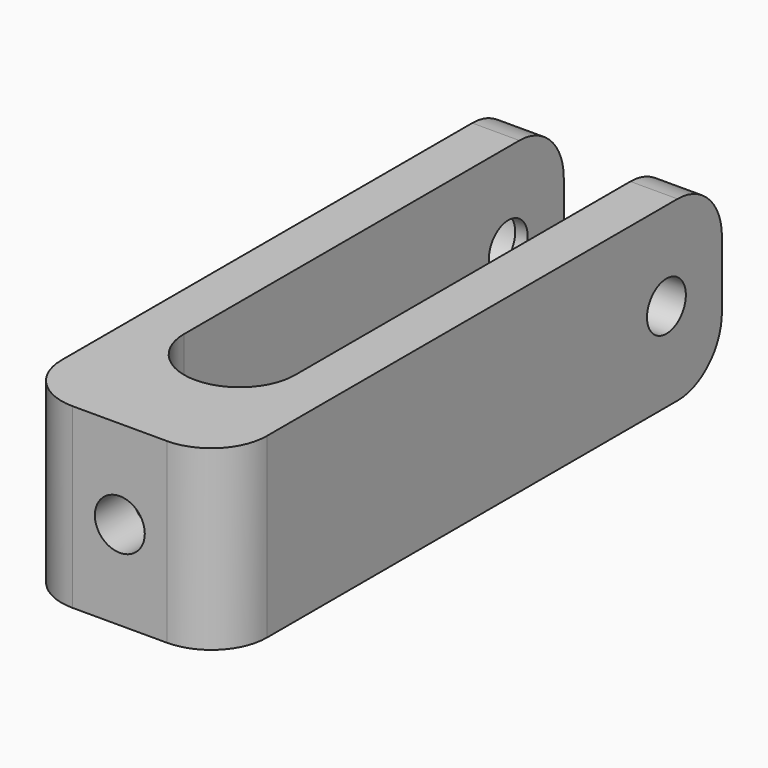
from build123d import *

# Parameters (mm, degrees)
F0_W         = 3.4
F0_H         = 12.8
F0_W_2       = 8
F0_R         = 1.8
F1_DEPTH     = 45
F2_R         = 1.75
F3_DEPTH     = 25
F2_R_2       = 3
F4_DEPTH     = 2.5
F0_H_2       = 0.6
F5_DEPTH     = 38.2
F6_T3_DEPTH  = 12.8
F6_S4_R      = 1.8
F6_T5_DEPTH  = 8
F6_T8_DEPTH  = 12.8
F6_S9_R      = 1.8
F6_T10_DEPTH = 8
F6_T14_DEPTH = 23.4
F6_T17_DEPTH = 23.4
F6_T20_DEPTH = 23.4
F6_T23_DEPTH = 23.4
F6_T26_DEPTH = 32.8
F6_T29_DEPTH = 32.8
F7_DEPTH     = 41.6


# Not quite as in the source:
# - a fillet or chamfer that OpenCascade refuses, or shapes differently, is made with other operations: its cross-section is extruded or revolved along the edge and cut away or added


with BuildPart() as f1:
    # F0 (on Front) → F1 (new body)
    with BuildSketch(Plane.XZ):
        with Locations((-1.7, 6.4)):
            Rectangle(F0_W, F0_H)
        with Locations((-7.4, 6.4)):
            Rectangle(F0_W_2, F0_H)
        Polygon((-10.8641016151, 6.4), (-9.1320508076, 9.4), (-5.6679491924, 9.4), (-3.9358983849, 6.4), (-5.6679491924, 3.4), (-9.1320508076, 3.4), align=None, mode=Mode.SUBTRACT)
        with Locations((-13.1, 6.4)):
            Rectangle(F0_W, F0_H)
        Polygon((-5.6679491924, 9.4), (-9.1320508076, 9.4), (-10.8641016151, 6.4), (-9.1320508076, 3.4), (-5.6679491924, 3.4), (-3.9358983849, 6.4), align=None)
        with Locations((-7.4, 6.4)):
            Circle(F0_R, mode=Mode.SUBTRACT)
    extrude(amount=F1_DEPTH)

    # F2 (on face) → F3 (cut)
    with BuildSketch(Plane(origin=(-14.8, 0, 0), x_dir=(0, -1, 0), z_dir=(-1, 0, 0))):
        with Locations((5, 6.4)):
            Circle(F2_R)
    extrude(amount=-F3_DEPTH, mode=Mode.SUBTRACT)

    # F2 (on face) → F4 (cut)
    with BuildSketch(Plane(origin=(-14.8, 0, 0), x_dir=(0, -1, 0), z_dir=(-1, 0, 0))):
        with Locations((5, 6.4)):
            Circle(F2_R_2)
        with Locations((5, 6.4)):
            Circle(F2_R, mode=Mode.SUBTRACT)
    extrude(amount=-F4_DEPTH, mode=Mode.SUBTRACT)

    # F0 (on Front) → F5 (cut)
    with BuildSketch(Plane.XZ):
        with Locations((-7.4, 13.1)):
            Rectangle(F0_W_2, F0_H_2)
        with Locations((-7.4, 6.4)):
            Rectangle(F0_W_2, F0_H)
        Polygon((-10.8641016151, 6.4), (-9.1320508076, 9.4), (-5.6679491924, 9.4), (-3.9358983849, 6.4), (-5.6679491924, 3.4), (-9.1320508076, 3.4), align=None, mode=Mode.SUBTRACT)
        with Locations((-7.4, -0.3)):
            Rectangle(F0_W_2, F0_H_2)
        Polygon((-5.6679491924, 9.4), (-9.1320508076, 9.4), (-10.8641016151, 6.4), (-9.1320508076, 3.4), (-5.6679491924, 3.4), (-3.9358983849, 6.4), align=None)
        with Locations((-7.4, 6.4)):
            Circle(F0_R, mode=Mode.SUBTRACT)
    extrude(amount=F5_DEPTH, mode=Mode.SUBTRACT)

    # F6: fillet of radius 4 on 8 edges, made by hand


with BuildPart() as f6_tool1:
    # F6_s2 → F6_t3 (new body)
    with BuildSketch(Plane.XY):
        with BuildLine():
            ThreePointArc((-7.4, -38.2), (-4.5715728753, -37.0284271247), (-3.4, -34.2))
            Line((-3.4, -34.2), (-3.4, -38.2))
            Line((-3.4, -38.2), (-7.4, -38.2))
        make_face()
    extrude(amount=F6_T3_DEPTH)

    # F6_s4 → F6_t5 (cut, symmetric)
    with BuildSketch(Plane.XZ.offset(36.2)):
        with Locations((-7.4, 6.4)):
            Circle(F6_S4_R)
    extrude(amount=F6_T5_DEPTH, both=True, mode=Mode.SUBTRACT)


with BuildPart() as f6_tool6:
    # F6_s7 → F6_t8 (new body)
    with BuildSketch(Plane.XY.offset(12.8)):
        with BuildLine():
            ThreePointArc((-11.4, -34.2), (-10.2284271247, -37.0284271247), (-7.4, -38.2))
            Line((-7.4, -38.2), (-11.4, -38.2))
            Line((-11.4, -38.2), (-11.4, -34.2))
        make_face()
    extrude(amount=-F6_T8_DEPTH)

    # F6_s9 → F6_t10 (cut, symmetric)
    with BuildSketch(Plane.XZ.offset(36.2)):
        with Locations((-7.4, 6.4)):
            Circle(F6_S9_R)
    extrude(amount=F6_T10_DEPTH, both=True, mode=Mode.SUBTRACT)


with BuildPart() as f1_1:
    add(f1.part)

    # F6_t11: union F6_tool1, F6_tool6
    add([f6_tool1.part, f6_tool6.part])


with BuildPart() as f6_tool12:
    # F6_s13 → F6_t14 (new body)
    with BuildSketch(Plane.YZ.offset(10)):
        with BuildLine():
            ThreePointArc((0, 8.8), (-1.1715728753, 11.6284271247), (-4, 12.8))
            Line((-4, 12.8), (0, 12.8))
            Line((0, 12.8), (0, 8.8))
        make_face()
    extrude(amount=-F6_T14_DEPTH)


with BuildPart() as f6_tool15:
    # F6_s16 → F6_t17 (new body)
    with BuildSketch(Plane.YZ.offset(-13.4)):
        with BuildLine():
            ThreePointArc((-4, 0), (-1.1715728753, 1.1715728753), (0, 4))
            Line((0, 4), (0, 0))
            Line((0, 0), (-4, 0))
        make_face()
    extrude(amount=F6_T17_DEPTH)


with BuildPart() as f6_tool18:
    # F6_s19 → F6_t20 (new body)
    with BuildSketch(Plane.YZ.offset(-24.8)):
        with BuildLine():
            ThreePointArc((-4, 0), (-1.1715728753, 1.1715728753), (0, 4))
            Line((0, 4), (0, 0))
            Line((0, 0), (-4, 0))
        make_face()
    extrude(amount=F6_T20_DEPTH)


with BuildPart() as f6_tool21:
    # F6_s22 → F6_t23 (new body)
    with BuildSketch(Plane.YZ.offset(-1.4)):
        with BuildLine():
            ThreePointArc((-4, 12.8), (-1.1715728753, 11.6284271247), (0, 8.8))
            Line((0, 8.8), (0, 12.8))
            Line((0, 12.8), (-4, 12.8))
        make_face()
    extrude(amount=-F6_T23_DEPTH)


with BuildPart() as f6_tool24:
    # F6_s25 → F6_t26 (new body)
    with BuildSketch(Plane.XY.offset(22.8)):
        with BuildLine():
            ThreePointArc((-10.8, -45), (-13.6284271247, -43.8284271247), (-14.8, -41))
            Line((-14.8, -41), (-14.8, -45))
            Line((-14.8, -45), (-10.8, -45))
        make_face()
    extrude(amount=-F6_T26_DEPTH)


with BuildPart() as f6_tool27:
    # F6_s28 → F6_t29 (new body)
    with BuildSketch(Plane.XY.offset(-10)):
        with BuildLine():
            ThreePointArc((0, -41), (-1.1715728753, -43.8284271247), (-4, -45))
            Line((-4, -45), (0, -45))
            Line((0, -45), (0, -41))
        make_face()
    extrude(amount=F6_T29_DEPTH)


with BuildPart() as f1_2:
    add(f1_1.part)

    # F6_t30: cut F6_tool12, F6_tool15, F6_tool18, F6_tool21, F6_tool24, F6_tool27
    add([f6_tool12.part, f6_tool15.part, f6_tool18.part, f6_tool21.part, f6_tool24.part, f6_tool27.part], mode=Mode.SUBTRACT)

    # F0 (on Front) → F7 (cut)
    with BuildSketch(Plane.XZ):
        Polygon((-5.6679491924, 9.4), (-9.1320508076, 9.4), (-10.8641016151, 6.4), (-9.1320508076, 3.4), (-5.6679491924, 3.4), (-3.9358983849, 6.4), align=None)
        with Locations((-7.4, 6.4)):
            Circle(F0_R, mode=Mode.SUBTRACT)
    extrude(amount=F7_DEPTH, mode=Mode.SUBTRACT)


solid = f1_2.part
